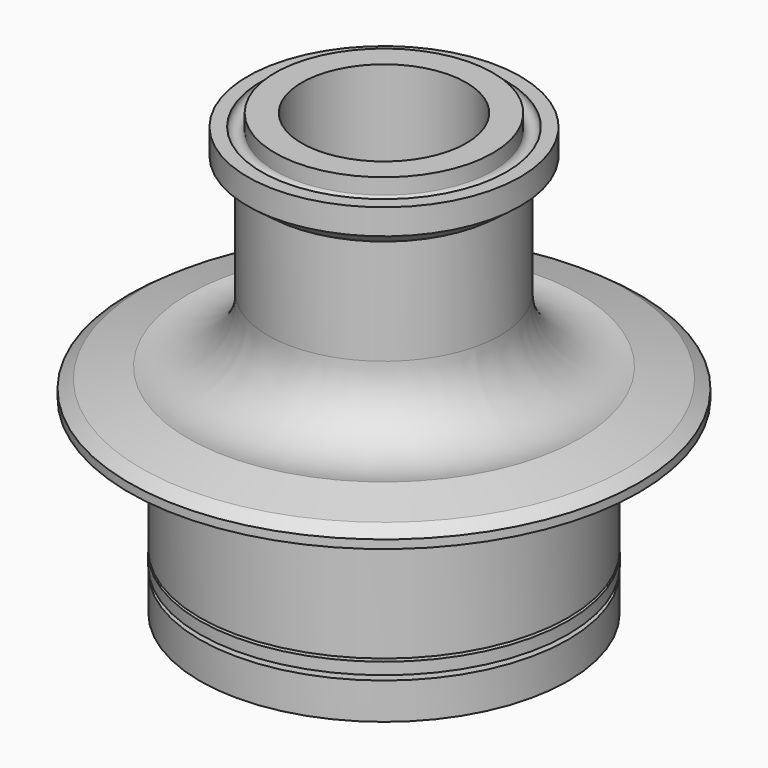
from build123d import *


with BuildPart() as f1:
    # F0 (on Front) → F1 (revolve)
    with BuildSketch(Plane.XZ):
        with BuildLine():
            Line((12.2577650473, 26.3742990792), (9.2577650473, 26.3742990792))
            Line((9.2577650473, 26.3742990792), (9.2577650473, -23.2081070539))
            Line((9.2577650473, -23.2081070539), (10.9627645774, -23.2081070539))
            add(Edge.make_bspline(
                [(19.8231283575, -23.2172738761), (18.0998597904, -21.8676731785), (15.286414199, -19.6408866692), (12.3874015782, -20.0680284116), (11.9609542206, -21.6848471621), (11.0441603331, -22.6479024969), (10.9627645774, -23.2081070539)],
                knots=[0, 0, 0, 0, 0.3730849217, 0.6049066924, 0.7930806457, 1, 1, 1, 1], degree=3))
            Line((19.8231283575, -23.2172738761), (20.7255259156, -23.2172738761))
            Line((20.7255259156, -23.2172738761), (20.7255259156, -19.1191080958))
            Line((20.7255259156, -19.1191080958), (19.4651619299, -19.1191080958))
            Line((19.4651619299, -19.1191080958), (19.4651619299, -18.5812935233))
            Line((19.4651619299, -18.5812935233), (20.7406301051, -18.5812935233))
            Line((20.7406301051, -18.5812935233), (20.7406301051, -17.2449033707))
            Line((20.7406301051, -17.2449033707), (20.0231876224, -17.2286070883))
            Line((20.0231876224, -17.2286070883), (20.0231876224, -16.9337423263))
            Line((20.0231876224, -16.9337423263), (20.7312413867, -16.9337423263))
            Line((20.7312413867, -16.9337423263), (20.7312413867, -3.6812480424))
            Line((20.7312413867, -3.6812480424), (22.978738881, -3.6812480424))
            Line((22.978738881, -3.6812480424), (22.978738881, -1.994405834))
            Line((22.978738881, -1.994405834), (24.7187081645, -1.994405834))
            ThreePointArc((24.7187081645, -1.994405834), (26.1406309916, -0.8455250202), (27.6167804076, -1.923845266))
            Line((27.6167804076, -1.923845266), (28.7137379414, -1.923845266))
            Line((28.7137379414, -1.923845266), (28.7137379414, -0.9687495106))
            Line((28.7137379414, -0.9687495106), (27.3187366885, 0))
            Line((27.3187366885, 0), (22.0342594068, 1.2435050098))
            ThreePointArc((22.0342594068, 1.2435050098), (15.7506244054, 2.6845196535), (13.0835622549, 8.5537079722))
            Line((13.0835622549, 8.5537079722), (13.0835622549, 20.4233584418))
            Line((13.0835622549, 20.4233584418), (15.3540684308, 22.1262395074))
            Line((15.3540684308, 22.1262395074), (15.3540684308, 25.0082887529))
            Line((15.3540684308, 25.0082887529), (13.8040684308, 25.0082887529))
            ThreePointArc((13.8040684308, 25.0082887529), (13.2300100677, 24.0508773646), (12.2577650473, 24.5994383828))
            Line((12.2577650473, 24.5994383828), (12.2577650473, 26.3742990792))
        make_face()
    revolve(axis=Axis((0, 0, -2.302121371), (0, 0, -1)))


solid = f1.part
